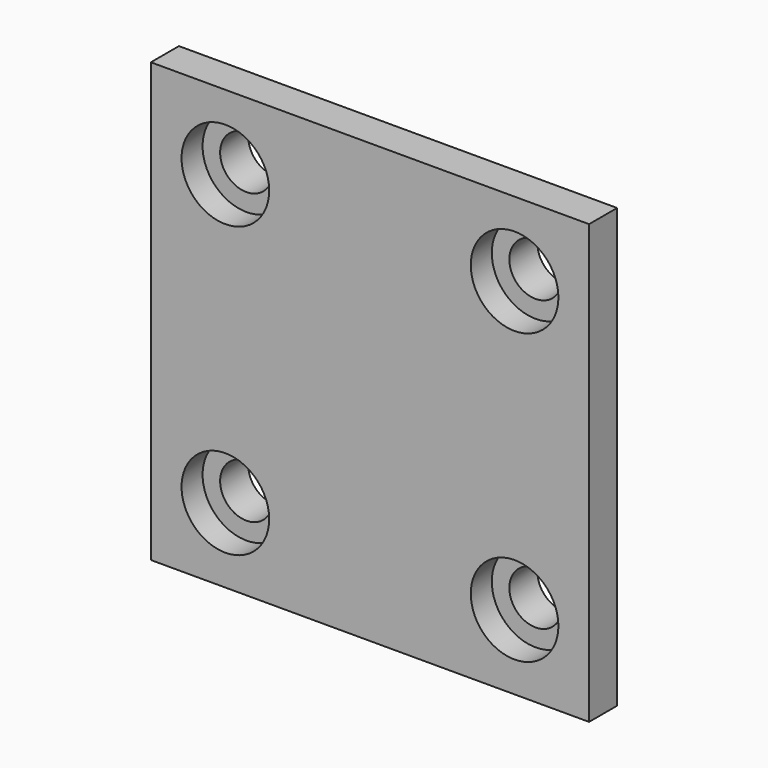
from build123d import *

# Parameters (mm, degrees)
F0_W     = 50
F0_H     = 50
F1_DEPTH = 4
F2_W     = 43.4
F2_H     = 43.4
F3_DEPTH = 3
F4_R     = 3
F5_DEPTH = 25
F6_R     = 5
F6_R_2   = 3
F7_DEPTH = 3
F8_R     = 3


# Not quite as in the source:
# - a feature names something its author has since deleted; it is built from what else it names


with BuildPart() as f1:
    # F0 (on Front) → F1 (new body)
    with BuildSketch(Plane.XZ):
        Rectangle(F0_W, F0_H)
    extrude(amount=-F1_DEPTH)

    # F2 (on face) → F3 (join)
    with BuildSketch(Plane(origin=(0, 4, 0), x_dir=(-1, 0, 0), z_dir=(0, 1, 0))):
        Rectangle(F2_W, F2_H)
    extrude(amount=F3_DEPTH)

    # F4 (on face) → F5 (cut)
    with BuildSketch(Plane(origin=(0, 7, 0), x_dir=(-1, 0, 0), z_dir=(0, 1, 0))):
        with Locations((-16.5, 16.5)):
            Circle(F4_R)
        with Locations((16.5, 16.5)):
            Circle(F4_R)
        with Locations((16.5, -16.5)):
            Circle(F4_R)
        with Locations((-16.5, -16.5)):
            Circle(F4_R)
    extrude(amount=-F5_DEPTH, mode=Mode.SUBTRACT)

    # F6 (on face) → F7 (cut)
    with BuildSketch(Plane.XZ):
        with Locations((-16.5, 16.5)):
            Circle(F6_R)
        with Locations((-16.5, 16.5)):
            Circle(F6_R_2, mode=Mode.SUBTRACT)
        with Locations((16.5, 16.5)):
            Circle(F6_R)
        with Locations((16.5, 16.5)):
            Circle(F6_R_2, mode=Mode.SUBTRACT)
        with Locations((16.5, -16.5)):
            Circle(F6_R)
        with Locations((16.5, -16.5)):
            Circle(F6_R_2, mode=Mode.SUBTRACT)
        with Locations((-16.5, -16.5)):
            Circle(F6_R)
        with Locations((-16.5, -16.5)):
            Circle(F6_R_2, mode=Mode.SUBTRACT)
    extrude(amount=-F7_DEPTH, mode=Mode.SUBTRACT)

    # F8
    f8_edges = [f1.edges().sort_by_distance(p)[0] for p in [
        (21.7, 5.5, 21.7),
        (-21.7, 5.5, 21.7),
        (-21.7, 5.5, -21.7),
        (21.7, 5.5, -21.7),
    ]]
    fillet(f8_edges, radius=F8_R)


solid = f1.part
